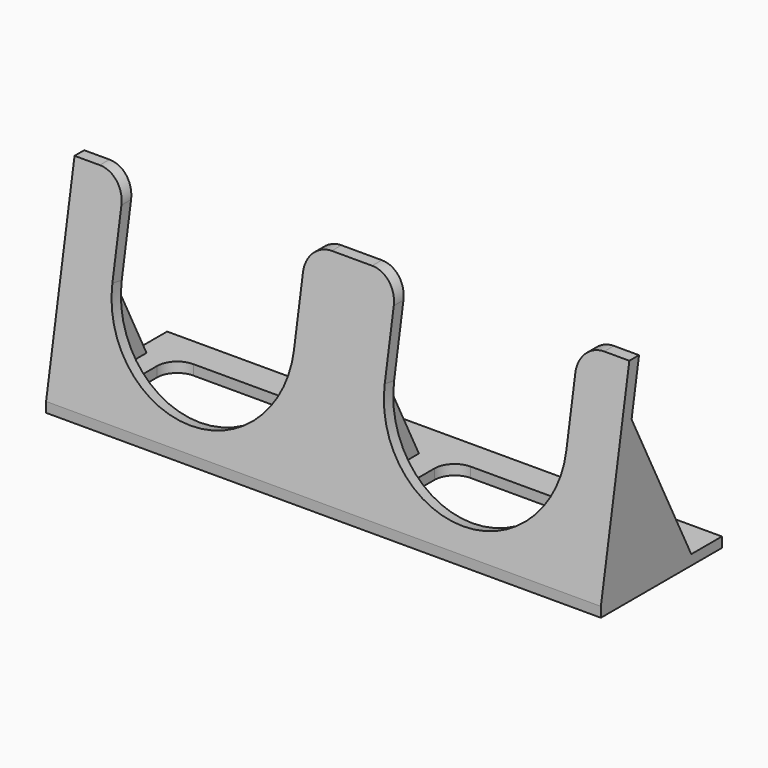
from build123d import *

# Parameters (mm, degrees)
F0_W         = 110
F0_H         = 30
F1_DEPTH     = 2
F3_DEPTH     = 55
F5_DEPTH     = 2.3635386072
F7_DEPTH     = 2
F9_DEPTH     = 1
F10_W        = 43
F10_H        = 15.6
F11_DEPTH    = 2
F12_T1_DEPTH = 27.4
F13_R        = 4


# Not quite as in the source:
# - a fillet or chamfer that OpenCascade refuses, or shapes differently, is made with other operations: its cross-section is extruded or revolved along the edge and cut away or added
# - a pattern or mirror of a feature is missing from the dataset's text; its kind, count and spacing are read off the source's solid


with BuildPart() as f1:
    # F0 (on Top) → F1 (new body)
    with BuildSketch(Plane.XY):
        Rectangle(F0_W, F0_H)
    extrude(amount=F1_DEPTH)

    # F2 (on Right) → F3 (join, symmetric)
    with BuildSketch(Plane.YZ):
        Polygon((-15, 2), (-12.6, 2), (-5.5469207717, 42), (-7.9469207717, 42), align=None)
    extrude(amount=F3_DEPTH, both=True)

    # F4 (on face) → F5 (cut, through all)
    with BuildSketch(Plane(origin=(0, -14.8897147992, 2.6254584542), x_dir=(1, 0, 0), z_dir=(0, -0.984807753, 0.1736481777))):
        with BuildLine():
            Line((-9, 21.9819573165), (-9, 39.9819573165))
            Line((-9, 39.9819573165), (-9, 44.9819573165))
            Line((-9, 44.9819573165), (-45, 44.9819573165))
            Line((-45, 44.9819573165), (-45, 39.9819573165))
            Line((-45, 39.9819573165), (-45, 21.9819573165))
            ThreePointArc((-45, 21.9819573165), (-27, 3.9819573165), (-9, 21.9819573165))
        make_face()
    f5 = extrude(amount=-F5_DEPTH, mode=Mode.SUBTRACT)

    # F5_copies: F5 across plane
    add(f5.mirror(Plane(origin=(0, 0, 0), x_dir=(0, 0, 1), z_dir=(1, 0, 0))), mode=Mode.SUBTRACT)

    # F6 (on face) → F7 (join)
    with BuildSketch(Plane(origin=(-55, 0, 0), x_dir=(0, -1, 0), z_dir=(-1, 0, 0))):
        Polygon((7.39055467, 31.5442325904), (-7.4, 2), (12.6, 2), align=None)
    f7 = extrude(amount=-F7_DEPTH)

    # F7_copies: F7 across plane
    add(f7.mirror(Plane(origin=(0, 0, 0), x_dir=(0, 0, 1), z_dir=(1, 0, 0))))

    # F8 (on Right) → F9 (join, symmetric)
    with BuildSketch(Plane.YZ):
        Polygon((-12.6, 2), (7.4, 2), (-7.39055467, 31.5442325904), align=None)
    extrude(amount=F9_DEPTH, both=True)

    # F10 (on Top) → F11 (cut, through all)
    with BuildSketch(Plane.XY):
        with Locations((27.5, 1.2)):
            Rectangle(F10_W, F10_H)
        with Locations((-27.5, 1.2)):
            Rectangle(F10_W, F10_H)
    extrude(amount=F11_DEPTH, mode=Mode.SUBTRACT)

    # F12: fillet of radius 5 on 6 edges, made by hand

    # F12_s2 → F12_t1 (cut)
    with BuildSketch(Plane.XZ.offset(-6.9530792283)):
        with BuildLine():
            ThreePointArc((50, 42), (46.4644660941, 40.5355339059), (45, 37))
            Line((45, 37), (45, 42))
            Line((45, 42), (50, 42))
        make_face()
        with BuildLine():
            ThreePointArc((-45, 37), (-46.4644660941, 40.5355339059), (-50, 42))
            Line((-50, 42), (-45, 42))
            Line((-45, 42), (-45, 37))
        make_face()
        with BuildLine():
            ThreePointArc((-9, 37), (-7.5355339059, 40.5355339059), (-4, 42))
            Line((-4, 42), (-9, 42))
            Line((-9, 42), (-9, 37))
        make_face()
        with BuildLine():
            ThreePointArc((4, 42), (7.5355339059, 40.5355339059), (9, 37))
            Line((9, 37), (9, 42))
            Line((9, 42), (4, 42))
        make_face()
    extrude(amount=F12_T1_DEPTH, mode=Mode.SUBTRACT)

    # F13
    f13_edges = [f1.edges().sort_by_distance(p)[0] for p in [
        (-49, -6.6, 1),
        (49, -6.6, 1),
        (-6, -6.6, 1),
        (6, -6.6, 1),
        (6, 9, 1),
        (-49, 9, 1),
        (49, 9, 1),
        (-6, 9, 1),
    ]]
    fillet(f13_edges, radius=F13_R)


solid = f1.part
